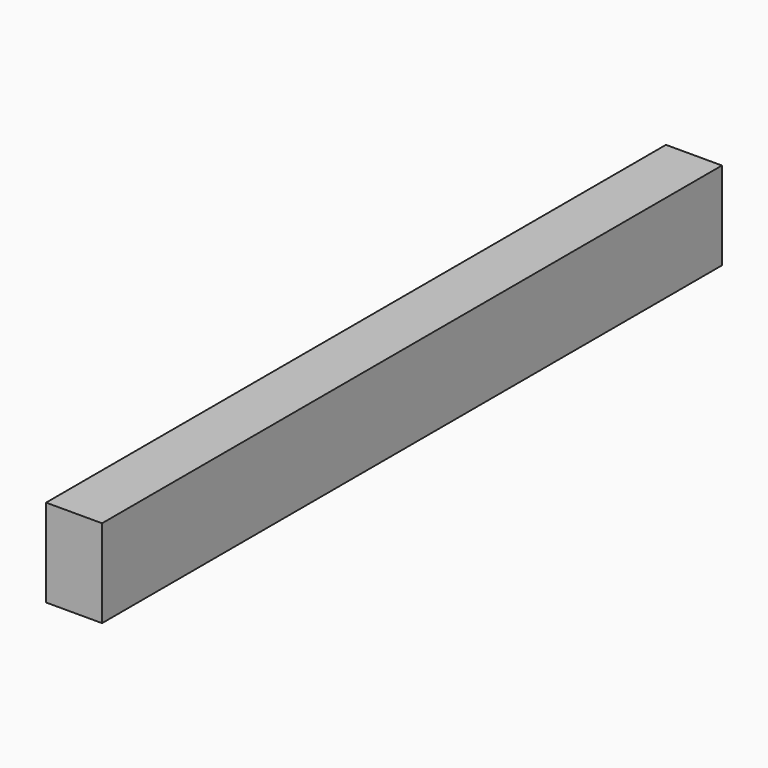
from build123d import *

# Parameters (mm, degrees)
F2_W     = 1.9140616059
F2_H     = 3.0078124255
F3_DEPTH = 25
F4_DEPTH = 0.65
F5_DEPTH = 0.85


# Not quite as in the source:
# - the program builds the solid bodies; features that only make, move or delete a surface that nothing else refers to are left out


with BuildPart() as f3:
    # F2 (on Front) → F3 (new body)
    with BuildSketch(Plane.XZ):
        with Locations((44.2285165191, 23.0371104553)):
            Rectangle(F2_W, F2_H)
    extrude(amount=F3_DEPTH)

    # F4 (add): a face of the model
    f4_faces = [f3.faces().sort_by_distance(p)[0] for p in [
        (44.2285165191, 0, 23.0371104553),
    ]]
    extrude(f4_faces, amount=F4_DEPTH)

    # F5 (add): a face of the model
    f5_faces = [f3.faces().sort_by_distance(p)[0] for p in [
        (44.2285165191, -25, 23.0371104553),
    ]]
    extrude(f5_faces, amount=F5_DEPTH)


solid = f3.part
